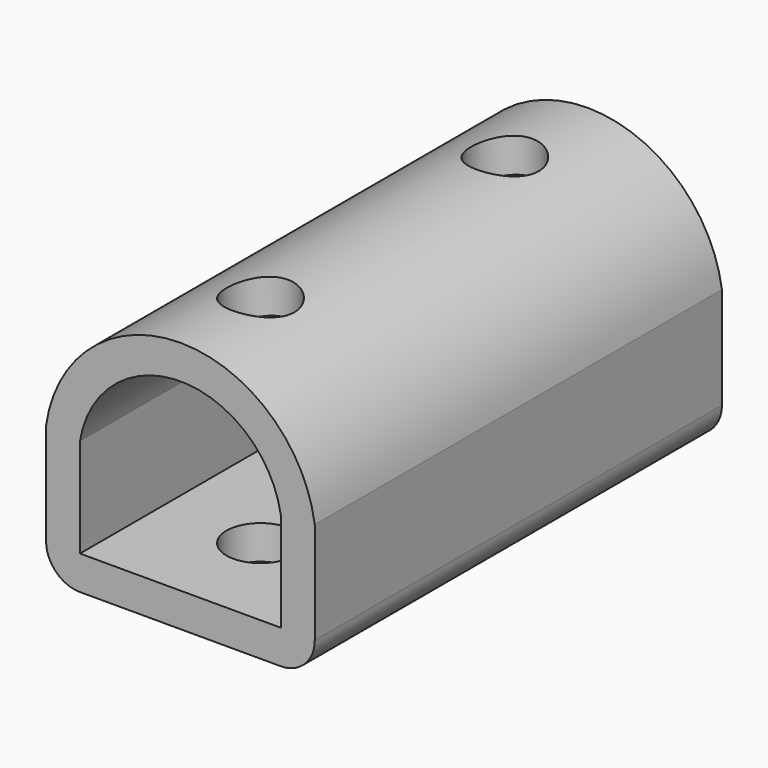
from build123d import *

# Parameters (mm, degrees)
F1_DEPTH = 75
F3_DEPTH = 75.001
F4_R     = 5
F5_DEPTH = 37.1620739384
F6_R     = 5


# Not quite as in the source:
# - a feature of the source that left no trace in its solid (it failed there, or was rolled back) is left out


with BuildPart() as f1:
    # F0 (on Front) → F1 (new body)
    with BuildSketch(Plane.XZ):
        with BuildLine():
            ThreePointArc((39.5949743688, 20), (19.7974871844, 37.1610739384), (0, 20))
            Line((0, 20), (0, 0))
            Line((0, 0), (39.5949743688, 0))
            Line((39.5949743688, 0), (39.5949743688, 20))
        make_face()
    extrude(amount=F1_DEPTH)

    # F2 (on face) → F3 (cut, through all)
    with BuildSketch(Plane.XZ.offset(75)):
        with BuildLine():
            Line((34.5949743688, 5), (34.5949743688, 19.6175700258))
            ThreePointArc((34.5949743688, 19.6175700258), (19.7974871844, 32.1610739384), (5, 19.6175700258))
            Line((5, 19.6175700258), (5, 5))
            Line((5, 5), (34.5949743688, 5))
        make_face()
    extrude(amount=-F3_DEPTH, mode=Mode.SUBTRACT)

    # F4 (on face) → F5 (cut, through all)
    with BuildSketch(Plane(origin=(0, 0, 0), x_dir=(1, 0, 0), z_dir=(0, 0, -1))):
        with Locations((19.5949743688, 60)):
            Circle(F4_R)
        with Locations((19.5949743688, 15)):
            Circle(F4_R)
    extrude(amount=-F5_DEPTH, mode=Mode.SUBTRACT)

    # F6
    f6_edges = [f1.edges().sort_by_distance(p)[0] for p in [
        (39.594974, -37.5, 0),
        (0, -37.5, 0),
    ]]
    fillet(f6_edges, radius=F6_R)


solid = f1.part
